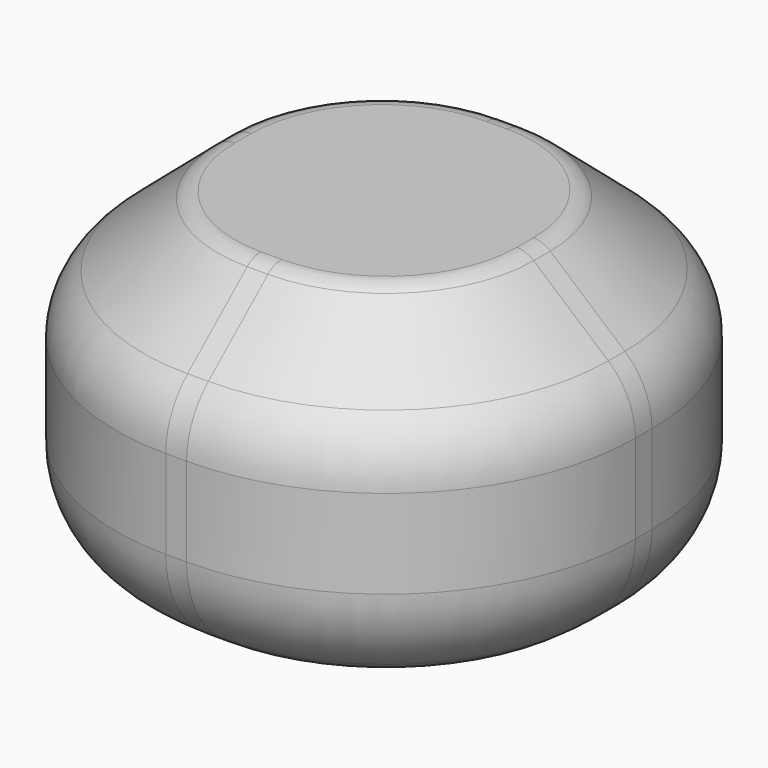
from build123d import *

# Parameters (mm, degrees)
F3_DEPTH  = 0.4
F4_DEPTH  = 0.65
F5_ANGLE  = 90
F9_ANGLE  = -90
F11_ANGLE = 180
F13_DEPTH = 0.6
F14_R     = 0.1675
F17_DEPTH = 0.1


# Not quite as in the source:
# - a feature of the source that left no trace in its solid (it failed there, or was rolled back) is left out


with BuildPart() as f3:
    # F2 (on Front) → F3 (new body)
    with BuildSketch(Plane.XZ):
        with BuildLine():
            Line((0, 0.3), (0, 0))
            Line((0, 0), (3.6876645899, 0))
            ThreePointArc((3.6876645899, 0), (3.7184315179, 0.004850664), (3.7462136453, 0.0189320772))
            Line((3.7462136453, 0.0189320772), (3.9709811077, 0.1812641333))
            ThreePointArc((3.9709811077, 0.1812641333), (4.5807248826, 0.8921178442), (4.8, 1.8026225901))
            Line((4.8, 1.8026225901), (4.8, 3.5100976163))
            ThreePointArc((4.8, 3.5100976163), (4.6627693477, 4.1368828306), (4.2761870602, 4.6489825198))
            Line((4.2761870602, 4.6489825198), (2.8404336486, 5.8796283012))
            ThreePointArc((2.8404336486, 5.8796283012), (2.6885110858, 5.9689425075), (2.5150379619, 6))
            Line((2.5150379619, 6), (0, 6))
            Line((0, 6), (0, 5.55))
            Line((0, 5.55), (2.5733712952, 5.55))
            ThreePointArc((2.5733712952, 5.55), (2.60806592, 5.5437885015), (2.6384504326, 5.5259256602))
            Line((2.6384504326, 5.5259256602), (4.0158705108, 4.3452798789))
            ThreePointArc((4.0158705108, 4.3452798789), (4.2993641883, 3.9697401068), (4.4, 3.5100976163))
            Line((4.4, 3.5100976163), (4.4, 1.812848816))
            ThreePointArc((4.4, 1.812848816), (4.2223871549, 1.0753399719), (3.7284946972, 0.499548466))
            Line((3.7284946972, 0.499548466), (3.4521968212, 0.3))
            Line((3.4521968212, 0.3), (0, 0.3))
        make_face()
    extrude(amount=F3_DEPTH)

    # F4 (add): a face of the model
    f4_faces = [f3.faces().sort_by_distance(p)[0] for p in [
        (0, -0.2, 5.775),
    ]]
    extrude(f4_faces, amount=F4_DEPTH)

    # F2 (on Front) → F5 (revolve)
    with BuildSketch(Plane.XZ):
        with BuildLine():
            Line((0, 0.3), (0, 0))
            Line((0, 0), (3.6876645899, 0))
            ThreePointArc((3.6876645899, 0), (3.7184315179, 0.004850664), (3.7462136453, 0.0189320772))
            Line((3.7462136453, 0.0189320772), (3.9709811077, 0.1812641333))
            ThreePointArc((3.9709811077, 0.1812641333), (4.5807248826, 0.8921178442), (4.8, 1.8026225901))
            Line((4.8, 1.8026225901), (4.8, 3.5100976163))
            ThreePointArc((4.8, 3.5100976163), (4.6627693477, 4.1368828306), (4.2761870602, 4.6489825198))
            Line((4.2761870602, 4.6489825198), (2.8404336486, 5.8796283012))
            ThreePointArc((2.8404336486, 5.8796283012), (2.6885110858, 5.9689425075), (2.5150379619, 6))
            Line((2.5150379619, 6), (0, 6))
            Line((0, 6), (0, 5.55))
            Line((0, 5.55), (2.5733712952, 5.55))
            ThreePointArc((2.5733712952, 5.55), (2.60806592, 5.5437885015), (2.6384504326, 5.5259256602))
            Line((2.6384504326, 5.5259256602), (4.0158705108, 4.3452798789))
            ThreePointArc((4.0158705108, 4.3452798789), (4.2993641883, 3.9697401068), (4.4, 3.5100976163))
            Line((4.4, 3.5100976163), (4.4, 1.812848816))
            ThreePointArc((4.4, 1.812848816), (4.2223871549, 1.0753399719), (3.7284946972, 0.499548466))
            Line((3.7284946972, 0.499548466), (3.4521968212, 0.3))
            Line((3.4521968212, 0.3), (0, 0.3))
        make_face()
    revolve(axis=Axis((0, 0, 5.775), (0, 0, 1)), revolution_arc=F5_ANGLE)


with BuildPart() as f9_1:
    # F9: copy of F3
    add(f3.part.rotate(Axis((-0.2, -0.2, 0.1248804607), (0, 0, 1)), F9_ANGLE))


with BuildPart() as f3_1:
    add(f3.part)

    # F10: union F9_1
    add(f9_1.part)


with BuildPart() as f11_1:
    # F11: copy of F3
    add(f3_1.part.rotate(Axis((-0.2, -0.2, 0.1248804607), (0, 0, 1)), F11_ANGLE))


with BuildPart() as f3_2:
    add(f3_1.part)

    # F12: union F11_1
    add(f11_1.part)

    # F13 (add): a face of the model
    f13_faces = [f3_2.faces().sort_by_distance(p)[0] for p in [
        (-0.2, 0, 0.15),
    ]]
    extrude(f13_faces, amount=F13_DEPTH)

    # F14 (on face) → F17 (join)
    with BuildSketch(Plane(origin=(0, 0, 0), x_dir=(1, 0, 0), z_dir=(0, 0, -1))):
        Circle(F14_R)
    extrude(amount=F17_DEPTH)


solid = f3_2.part
